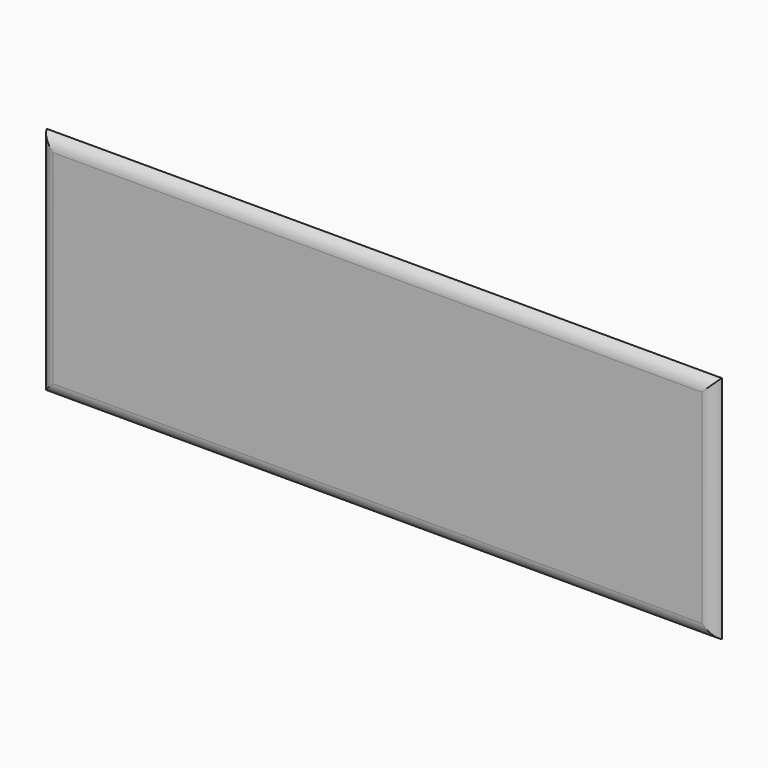
from build123d import *

# Parameters (mm, degrees)
F0_W        = 596.9
F0_H        = 203.2
F1_DEPTH    = 7.62
F2_T1_DEPTH = 655.0987113259
F2_T3_DEPTH = 261.3987113259


# Not quite as in the source:
# - a fillet or chamfer that OpenCascade refuses, or shapes differently, is made with other operations: its cross-section is extruded or revolved along the edge and cut away or added


with BuildPart() as f1:
    # F0 (on Front) → F1 (new body)
    with BuildSketch(Plane.XZ):
        with Locations((3.1592100859, 36.5264592544)):
            Rectangle(F0_W, F0_H)
    extrude(amount=F1_DEPTH)

    # F2: fillet of radius 12.7 on 4 edges, made by hand

    # F2_s2 → F2_t1 (cut)
    with BuildSketch(Plane.YZ.offset(-324.3901455771)):
        with BuildLine():
            ThreePointArc((0, 138.1264592544), (-5.545582337, 133.4427934696), (-7.62, 126.4867169893))
            Line((-7.62, 126.4867169893), (-7.62, 138.1264592544))
            Line((-7.62, 138.1264592544), (0, 138.1264592544))
        make_face()
        with BuildLine():
            ThreePointArc((0, -65.0735407456), (-5.545582337, -60.3898749607), (-7.62, -53.4337984804))
            Line((-7.62, -53.4337984804), (-7.62, -65.0735407456))
            Line((-7.62, -65.0735407456), (0, -65.0735407456))
        make_face()
    extrude(amount=F2_T1_DEPTH, mode=Mode.SUBTRACT)

    # F2_s4 → F2_t3 (cut)
    with BuildSketch(Plane.XY.offset(-94.1728964085)):
        with BuildLine():
            ThreePointArc((-295.2907899141, 0), (-290.6071241293, -5.545582337), (-283.6510476489, -7.62))
            Line((-283.6510476489, -7.62), (-295.2907899141, -7.62))
            Line((-295.2907899141, -7.62), (-295.2907899141, 0))
        make_face()
        with BuildLine():
            ThreePointArc((301.6092100859, 0), (296.925544301, -5.545582337), (289.9694678207, -7.62))
            Line((289.9694678207, -7.62), (301.6092100859, -7.62))
            Line((301.6092100859, -7.62), (301.6092100859, 0))
        make_face()
    extrude(amount=F2_T3_DEPTH, mode=Mode.SUBTRACT)


solid = f1.part
